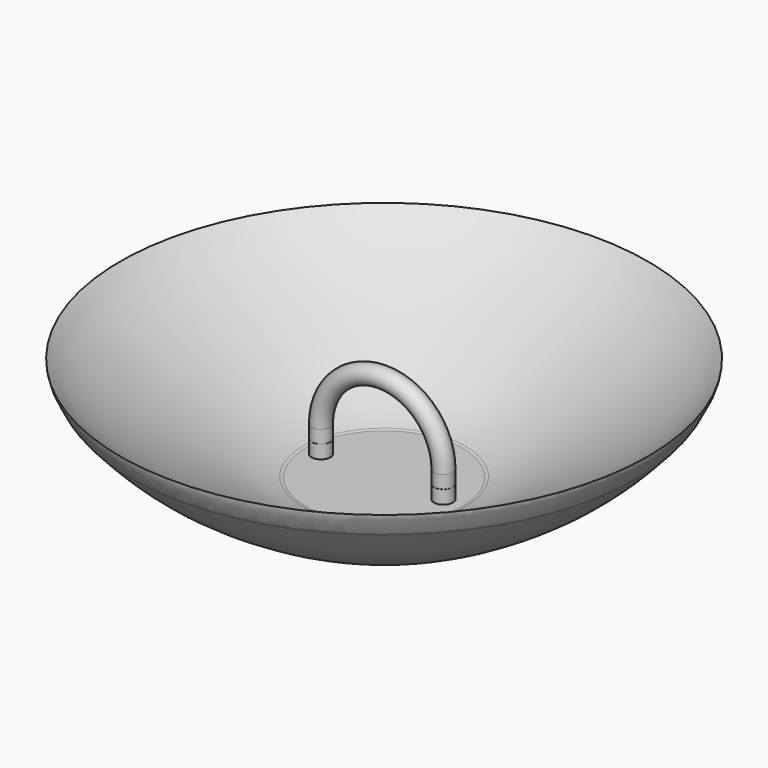
from build123d import *

# Parameters (mm, degrees)
F2_R     = 2.3237449832
F3_DEPTH = 3.302
F5_R     = 2.297710376


with BuildPart() as f1:
    # F0 (on Front) → F1 (revolve)
    with BuildSketch(Plane.XZ):
        with BuildLine():
            Line((0, 6.4537934959), (0, 0))
            add(Edge.make_bspline(
                [(0, 0), (5.3284348472, -0.151710014), (15.72935931, -0.4478428262), (29.3389014843, 1.9305018047), (51.2608661721, 14.7579911883), (58.4457571071, 22.5755026998), (61.4702167229, 25.9222669945)],
                knots=[0, 0, 0, 0, 0.2365448276, 0.4617274968, 0.7636676557, 0.990708621, 0.990708621, 0.990708621, 0.990708621], degree=3))
            add(Edge.make_bspline(
                [(61.4702167229, 25.9222669945), (61.5939891026, 26.0592293064), (61.7176621251, 26.1961773073), (61.8413351476, 26.3331253082)],
                knots=[0.990708621, 0.990708621, 0.990708621, 0.990708621, 1, 1, 1, 1], degree=3))
            add(Edge.make_bspline(
                [(19.9362844459, 6.6261832632), (23.0642313587, 6.9219216887), (33.6752694158, 9.3293914475), (61.2871102192, 26.430349091), (61.8413351476, 26.3331253082)],
                knots=[0.3055996998, 0.3055996998, 0.3055996998, 0.3055996998, 0.5203732934, 0.9456071412, 0.9456071412, 0.9456071412, 0.9456071412], degree=3))
            add(Edge.make_bspline(
                [(19.1792435944, 6.4537934959), (19.4312115798, 6.5108323155), (19.6831795651, 6.5678711352), (19.9362844459, 6.6261832632)],
                knots=[0, 0, 0, 0, 0.0222393359, 0.0222393359, 0.0222393359, 0.0222393359], degree=3))
            Line((19.1792435944, 6.4537934959), (16.7044717818, 6.4537934959))
            add(Edge.make_bspline(
                [(6.8562417291, 6.4537934959), (10.174427629, 6.4130106646), (13.4923483806, 6.3724655133), (16.7044717818, 6.4537934959)],
                knots=[0, 0, 0, 0, 0.2294042785, 0.2294042785, 0.2294042785, 0.2294042785], degree=3))
            Line((6.8562417291, 6.4537934959), (0, 6.4537934959))
        make_face()
        with BuildLine():
            add(Edge.make_bspline(
                [(19.9362844459, 6.6261832632), (23.0642313587, 6.9219216887), (33.6752694158, 9.3293914475), (61.2871102192, 26.430349091), (61.8413351476, 26.3331253082)],
                knots=[0.3055996998, 0.3055996998, 0.3055996998, 0.3055996998, 0.5203732934, 0.9456071412, 0.9456071412, 0.9456071412, 0.9456071412], degree=3))
            add(Edge.make_bspline(
                [(61.8413351476, 26.3331253082), (62.0067642507, 26.5338182356), (62.3784054543, 26.9846806276), (62.9694504555, 28.1334772092), (63.6191083309, 29.3888215381), (64.2996026431, 30.6889648721), (64.4545914573, 31.5078459617), (64.5285919309, 31.8988263607)],
                knots=[0, 0, 0, 0, 0.1633221476, 0.3669078679, 0.5840819466, 0.8014170695, 1, 1, 1, 1], degree=3))
            add(Edge.make_bspline(
                [(19.9362844459, 6.6261832632), (21.3897057398, 6.9610329441), (25.3615042434, 7.9649295402), (35.2978213246, 13.157404991), (48.0633763397, 19.7404571448), (59.9783712145, 27.3717771756), (63.2336508428, 30.610479627), (64.5285919309, 31.8988263607)],
                knots=[0.0222393359, 0.0222393359, 0.0222393359, 0.0222393359, 0.1499457799, 0.3624504838, 0.6085472144, 0.844281182, 1, 1, 1, 1], degree=3))
        make_face()
        with BuildLine():
            Line((16.7044717818, 6.4537934959), (6.8562417291, 6.4537934959))
            add(Edge.make_bspline(
                [(6.8562417291, 6.4537934959), (10.174427629, 6.4130106646), (13.4923483806, 6.3724655133), (16.7044717818, 6.4537934959)],
                knots=[0, 0, 0, 0, 0.2294042785, 0.2294042785, 0.2294042785, 0.2294042785], degree=3))
        make_face()
    revolve(axis=Axis((0, 0, 3.2268967479), (0, 0, -1)))

    # F2 (on face) → F3 (join)
    with BuildSketch(Plane.XY.offset(6.4537934959)):
        with Locations((14.5165240392, 0)):
            Circle(F2_R)
        with Locations((-15.4276872054, 0)):
            Circle(F2_R)
    extrude(amount=F3_DEPTH)

    # F6: sweep along a path in F4
    with BuildLine(Plane.XZ) as f6_path:
        Line((12.192779056, 9.7557934959), (12.192779056, 12.927793109))
        ThreePointArc((12.192779056, 12.927793109), (-0.4555815831, 25.5761537481), (-13.1039422222, 12.927793109))
        Line((-13.1039422222, 12.927793109), (-13.1039422222, 9.7557934959))
    # F5 (on face) → F6 (sweep)
    with BuildSketch(Plane.XY.offset(9.7557934959)):
        with Locations((14.5165240392, 0)):
            Circle(F5_R)
    sweep(path=f6_path.line)


solid = f1.part
